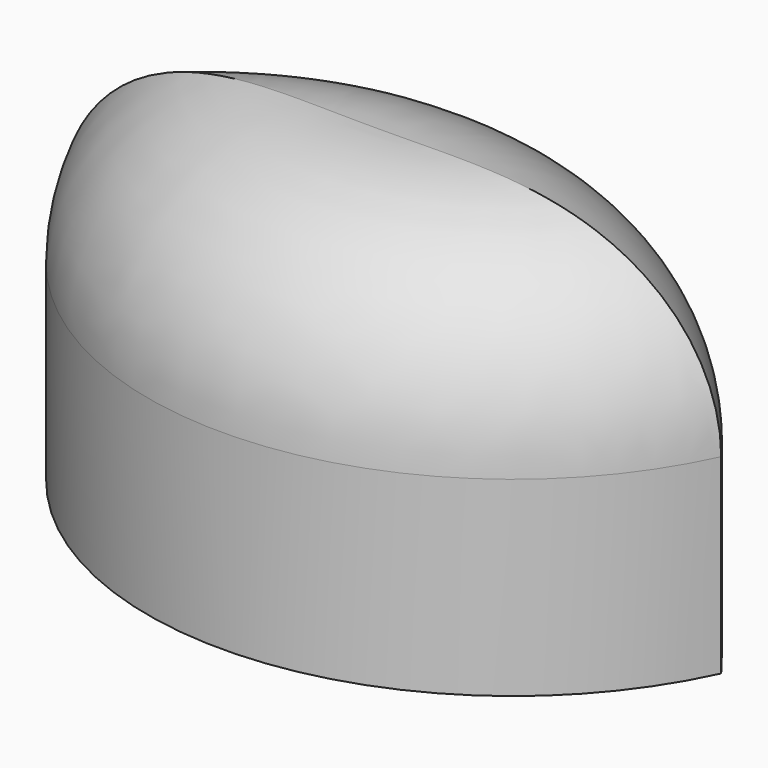
from build123d import *

# Parameters (mm, degrees)
F1_DEPTH    = 3
F2_T2_ANGLE = 243.5507728325
F2_T4_ANGLE = 280.4385461562


# Not quite as in the source:
# - a fillet or chamfer that OpenCascade refuses, or shapes differently, is made with other operations: its cross-section is extruded or revolved along the edge and cut away or added


with BuildPart() as f1:
    # F0 (on Top) → F1 (new body)
    with BuildSketch(Plane.XY):
        with BuildLine():
            ThreePointArc((-2.3295248933, 0), (0.2704751067, -1.6615556993), (2.8704751067, 0))
            ThreePointArc((2.8704751067, 0), (0.2704751067, 1.3384443007), (-2.3295248933, 0))
        make_face()
    extrude(amount=F1_DEPTH)

    # F2: fillet of radius 1.5 on 2 edges, made by hand

    # F2_s1 → F2_t2 (revolve, cut)
    with BuildSketch(Plane(origin=(-0.7559073156, -1.2203239289, 0), x_dir=(0, 0, 1), z_dir=(-0.5265906431, -0.8501189885, 0))):
        with BuildLine():
            ThreePointArc((1.5, -4.4018817505), (2.5606601718, -3.9625419223), (3, -2.9018817505))
            Line((3, -2.9018817505), (3, -4.4018817505))
            Line((3, -4.4018817505), (1.5, -4.4018817505))
        make_face()
    revolve(axis=Axis((0.2704751067, -1.856097729, 3), (0, 0, 1)), revolution_arc=F2_T2_ANGLE, mode=Mode.SUBTRACT)

    # F2_s3 → F2_t4 (revolve, cut)
    with BuildSketch(Plane(origin=(0.7515114026, 0.6257075418, 0), x_dir=(0, 0, 1), z_dir=(0.7684987994, 0.6398512291, 0))):
        with BuildLine():
            ThreePointArc((1.5, -3.6168099748), (2.5606601718, -3.1774701466), (3, -2.1168099748))
            Line((3, -2.1168099748), (3, -3.6168099748))
            Line((3, -3.6168099748), (1.5, -3.6168099748))
        make_face()
    revolve(axis=Axis((0.2704751067, 1.2034603053, 3), (0, 0, 1)), revolution_arc=F2_T4_ANGLE, mode=Mode.SUBTRACT)


solid = f1.part
